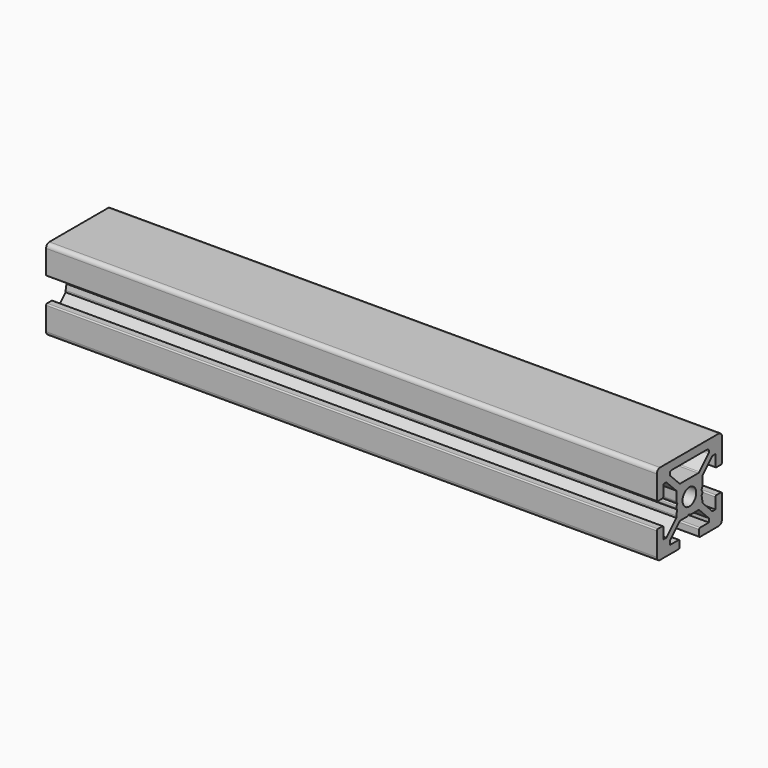
from build123d import *

# Parameters (mm, degrees)
F1_DEPTH = 75


# Not quite as in the source:
# - ends of sketch curves that miss each other by under 0.0002 mm in the source are joined


with BuildPart() as f1:
    # F0 (on Right) → F1 (new body, symmetric)
    with BuildSketch(Plane.YZ):
        with BuildLine():
            Line((9.043565, 10.073321), (0.043565, 10.073321))
            Line((0.043565, 10.073321), (-8.956435, 10.073321))
            ThreePointArc((-8.956435, 10.073321), (-9.6635417812, 9.7804277812), (-9.956435, 9.073321))
            Line((-9.956435, 9.073321), (-9.956435, 3.373321))
            ThreePointArc((-9.956435, 3.373321), (-9.8685670344, 3.1611889656), (-9.656435, 3.073321))
            Line((-9.656435, 3.073321), (-8.256435, 3.073321))
            ThreePointArc((-8.256435, 3.073321), (-8.0443029656, 3.1611889656), (-7.956435, 3.373321))
            Line((-7.956435, 3.373321), (-7.956435, 6.073321))
            Line((-7.956435, 6.073321), (-7.017095, 6.073321))
            Line((-7.017095, 6.073321), (-3.956435, 3.012661))
            Line((-3.956435, 3.012661), (-3.956435, 0.726911))
            ThreePointArc((-3.956435, 0.726911), (-3.9393979324, 0.5975015494), (-3.8894477764, 0.4769111291))
            Line((-3.8894477764, 0.4769111291), (-3.656435, 0.073321))
            Line((-3.656435, 0.073321), (-3.889448, -0.330269))
            ThreePointArc((-3.889448, -0.330269), (-3.956435, -0.580269), (-3.8894477764, -0.8302688709))
            Line((-3.8894477764, -0.8302688709), (-3.707412, -1.145565))
            Line((-3.707412, -1.145565), (-3.956435, -2.426679))
            Line((-3.956435, -2.426679), (-3.956435, -2.866019))
            Line((-3.956435, -2.866019), (-7.017095, -5.926679))
            Line((-7.017095, -5.926679), (-7.956435, -5.926679))
            Line((-7.956435, -5.926679), (-7.956435, -3.226679))
            ThreePointArc((-7.956435, -3.226679), (-8.0443029656, -3.0145469656), (-8.256435, -2.926679))
            Line((-8.256435, -2.926679), (-9.656435, -2.926679))
            ThreePointArc((-9.656435, -2.926679), (-9.8685670344, -3.0145469656), (-9.956435, -3.226679))
            Line((-9.956435, -3.226679), (-9.956435, -8.926679))
            ThreePointArc((-9.956435, -8.926679), (-9.6635417812, -9.6337857812), (-8.956435, -9.926679))
            Line((-8.956435, -9.926679), (-3.256435, -9.926679))
            ThreePointArc((-3.256435, -9.926679), (-3.0443029656, -9.8388110344), (-2.956435, -9.626679))
            Line((-2.956435, -9.626679), (-2.956435, -8.226679))
            ThreePointArc((-2.956435, -8.226679), (-3.0443029656, -8.0145469656), (-3.256435, -7.926679))
            Line((-3.256435, -7.926679), (-5.956435, -7.926679))
            Line((-5.956435, -7.926679), (-5.956435, -6.987339))
            Line((-5.956435, -6.987339), (-2.895775, -3.926679))
            Line((-2.895775, -3.926679), (-0.610025, -3.926679))
            ThreePointArc((-0.610025, -3.926679), (-0.4806155494, -3.9096419324), (-0.3600251291, -3.8596917764))
            Line((-0.3600251291, -3.8596917764), (-0.0645959325, -3.6891257984))
            Line((-0.0645959325, -3.6891257984), (0.2217128734, -3.8544264098))
            ThreePointArc((0.2217128734, -3.8544264098), (0.3921793907, -3.9150473077), (0.5730594828, -3.9110345539))
            ThreePointArc((0.5730594828, -3.9110345539), (0.6346161199, -3.9227524708), (0.697155, -3.926679))
            Line((0.697155, -3.926679), (2.982905, -3.926679))
            Line((2.982905, -3.926679), (6.043565, -6.987339))
            Line((6.043565, -6.987339), (6.043565, -7.926679))
            Line((6.043565, -7.926679), (3.343565, -7.926679))
            ThreePointArc((3.343565, -7.926679), (3.1314329656, -8.0145469656), (3.043565, -8.226679))
            Line((3.043565, -8.226679), (3.043565, -9.626679))
            ThreePointArc((3.043565, -9.626679), (3.1314329656, -9.8388110344), (3.343565, -9.926679))
            Line((3.343565, -9.926679), (9.043565, -9.926679))
            ThreePointArc((9.043565, -9.926679), (9.7506717812, -9.6337857812), (10.043565, -8.926679))
            Line((10.043565, -8.926679), (10.043565, -3.226679))
            ThreePointArc((10.043565, -3.226679), (9.9556970344, -3.0145469656), (9.743565, -2.926679))
            Line((9.743565, -2.926679), (8.343565, -2.926679))
            ThreePointArc((8.343565, -2.926679), (8.1314329656, -3.0145469656), (8.043565, -3.226679))
            Line((8.043565, -3.226679), (8.043565, -5.926679))
            Line((8.043565, -5.926679), (7.104225, -5.926679))
            Line((7.104225, -5.926679), (4.043565, -2.866019))
            Line((4.043565, -2.866019), (4.043565, -2.426679))
            Line((4.043565, -2.426679), (3.794542, -1.145565))
            Line((3.794542, -1.145565), (3.976578, -0.830269))
            ThreePointArc((3.976578, -0.830269), (4.043565, -0.580269), (3.9765777764, -0.3302691291))
            Line((3.9765777764, -0.3302691291), (3.743565, 0.073321))
            Line((3.743565, 0.073321), (3.976578, 0.476911))
            ThreePointArc((3.976578, 0.476911), (4.0265279324, 0.5975015494), (4.043565, 0.726911))
            Line((4.043565, 0.726911), (4.043565, 3.012661))
            Line((4.043565, 3.012661), (7.104225, 6.073321))
            Line((7.104225, 6.073321), (8.043565, 6.073321))
            Line((8.043565, 6.073321), (8.043565, 3.373321))
            ThreePointArc((8.043565, 3.373321), (8.1314329656, 3.1611889656), (8.343565, 3.073321))
            Line((8.343565, 3.073321), (9.743565, 3.073321))
            ThreePointArc((9.743565, 3.073321), (9.9556970344, 3.1611889656), (10.043565, 3.373321))
            Line((10.043565, 3.373321), (10.043565, 9.073321))
            ThreePointArc((10.043565, 9.073321), (9.7506717812, 9.7804277812), (9.043565, 10.073321))
        make_face()
        with BuildLine():
            ThreePointArc((0.043565, 2.173321), (2.143565, 0.073321), (0.043565, -2.026679))
            ThreePointArc((0.043565, -2.026679), (-2.056435, 0.073321), (0.043565, 2.173321))
        make_face(mode=Mode.SUBTRACT)
        with BuildLine():
            Line((2.775798, 4.073321), (0.043565, 4.073321))
            Line((0.043565, 4.073321), (-2.688668, 4.073321))
            ThreePointArc((-2.688668, 4.073321), (-2.8800097162, 4.1113812337), (-3.0422213906, 4.2197676094))
            Line((-3.0422213906, 4.2197676094), (-5.809988, 6.987535))
            ThreePointArc((-5.809988, 6.987535), (-5.9183747663, 7.1497462838), (-5.956435, 7.341088))
            Line((-5.956435, 7.341088), (-5.956435, 7.573321))
            ThreePointArc((-5.956435, 7.573321), (-5.8099883906, 7.9268743906), (-5.456435, 8.073321))
            Line((-5.456435, 8.073321), (0.043565, 8.073321))
            Line((0.043565, 8.073321), (5.543565, 8.073321))
            ThreePointArc((5.543565, 8.073321), (5.8971183906, 7.9268743906), (6.043565, 7.573321))
            Line((6.043565, 7.573321), (6.043565, 7.341088))
            ThreePointArc((6.043565, 7.341088), (6.0055047663, 7.1497462838), (5.8971183906, 6.9875346094))
            Line((5.8971183906, 6.9875346094), (3.129351, 4.219768))
            ThreePointArc((3.129351, 4.219768), (2.9671397162, 4.1113812337), (2.775798, 4.073321))
        make_face(mode=Mode.SUBTRACT)
    extrude(amount=F1_DEPTH, both=True)


solid = f1.part
